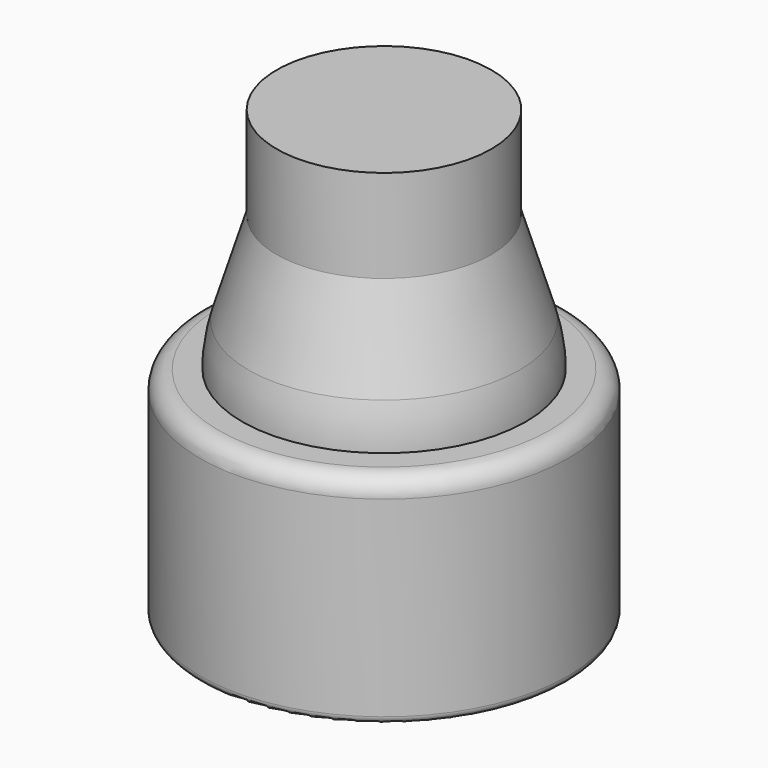
from build123d import *

# Parameters (mm, degrees)
F2_R     = 2.9977857905
F3_DEPTH = 5.85
F4_R     = 2.8
F5_DEPTH = 1
F5_TAPER = 70


# Not quite as in the source:
# - an extrude ends at something that could not be found from the text; its depth is read off the source's solid


with BuildPart() as f1:
    # F0 (on Front) → F1 (revolve)
    with BuildSketch(Plane.XZ):
        with BuildLine():
            Line((4.45, 5.85), (2.8, 5.85))
            Line((2.8, 5.85), (2.8, 3.65))
            Line((2.8, 3.65), (0.5, 2.3220943809))
            Line((0.5, 2.3220943809), (0, 2.3220943809))
            Line((0, 2.3220943809), (0, 0))
            Line((0, 0), (4.75, 0))
            ThreePointArc((4.75, 0), (4.8914213562, 0.0585786438), (4.95, 0.2))
            Line((4.95, 0.2), (4.95, 5.35))
            ThreePointArc((4.95, 5.35), (4.8035533906, 5.7035533906), (4.45, 5.85))
        make_face()
    revolve(axis=Axis((0, 0, 1.1610471904), (0, 0, -1)))

    # F2 (on face) → F3 (join, through all)
    with BuildSketch(Plane.XY.offset(5.85)):
        Circle(F2_R)
        with BuildLine():
            ThreePointArc((-0.5409184627, 2.3849386653), (0, 2.8), (0.5409184627, 2.3849386653))
            Line((0.5409184627, 2.3849386653), (0.5522855855, 2.3425159855))
            ThreePointArc((0.5522855855, 2.3425159855), (1.0088928953, 1.747453754), (1.7525355595, 1.6495513399))
            Line((1.7525355595, 1.6495513399), (1.7949582392, 1.6609184627))
            ThreePointArc((1.7949582392, 1.6609184627), (2.4248711306, 1.4), (2.3358767019, 0.7240202025))
            Line((2.3358767019, 0.7240202025), (2.304821145, 0.6929646456))
            ThreePointArc((2.304821145, 0.6929646456), (2.0177857905, 0), (2.304821145, -0.6929646456))
            Line((2.304821145, -0.6929646456), (2.3358767019, -0.7240202025))
            ThreePointArc((2.3358767019, -0.7240202025), (2.4248711306, -1.4), (1.7949582392, -1.6609184627))
            Line((1.7949582392, -1.6609184627), (1.7525355595, -1.6495513399))
            ThreePointArc((1.7525355595, -1.6495513399), (1.0088928953, -1.747453754), (0.5522855855, -2.3425159855))
            Line((0.5522855855, -2.3425159855), (0.5409184627, -2.3849386653))
            ThreePointArc((0.5409184627, -2.3849386653), (0, -2.8), (-0.5409184627, -2.3849386653))
            Line((-0.5409184627, -2.3849386653), (-0.5522855855, -2.3425159855))
            ThreePointArc((-0.5522855855, -2.3425159855), (-1.0088928953, -1.747453754), (-1.7525355595, -1.6495513399))
            Line((-1.7525355595, -1.6495513399), (-1.7949582392, -1.6609184627))
            ThreePointArc((-1.7949582392, -1.6609184627), (-2.4248711306, -1.4), (-2.3358767019, -0.7240202025))
            Line((-2.3358767019, -0.7240202025), (-2.304821145, -0.6929646456))
            ThreePointArc((-2.304821145, -0.6929646456), (-2.0177857905, 0), (-2.304821145, 0.6929646456))
            Line((-2.304821145, 0.6929646456), (-2.3358767019, 0.7240202025))
            ThreePointArc((-2.3358767019, 0.7240202025), (-2.4248711306, 1.4), (-1.7949582392, 1.6609184627))
            Line((-1.7949582392, 1.6609184627), (-1.7525355595, 1.6495513399))
            ThreePointArc((-1.7525355595, 1.6495513399), (-1.0088928953, 1.747453754), (-0.5522855855, 2.3425159855))
            Line((-0.5522855855, 2.3425159855), (-0.5409184627, 2.3849386653))
        make_face(mode=Mode.SUBTRACT)
    extrude(amount=-F3_DEPTH)

    # F4 (on face) → F5 (cut)
    with BuildSketch(Plane.XY.offset(5.85)):
        Circle(F4_R)
    extrude(amount=-F5_DEPTH, taper=F5_TAPER, mode=Mode.SUBTRACT)


with BuildPart() as f7:
    # F6 (on Front) → F7 (revolve)
    with BuildSketch(Plane.XZ):
        with BuildLine():
            Line((2.885, 12), (0, 12))
            Line((0, 12), (0, 0))
            Line((0, 0), (2.575, 0))
            Line((2.575, 0), (3.7168908213, 4.9460725434))
            ThreePointArc((3.7168908213, 4.9460725434), (3.8169738702, 5.9854747476), (3.644629586, 7.0153635796))
            Line((3.644629586, 7.0153635796), (2.885, 9.5))
            Line((2.885, 9.5), (2.885, 12))
        make_face()
    revolve(axis=Axis((0, 0, 6), (0, 0, -1)))


with BuildPart() as f9:
    # F8 (on Front) → F9 (revolve)
    with BuildSketch(Plane.XZ):
        with BuildLine():
            Line((0, 5.4649787367), (0, 0))
            Line((0, 0), (4.2405382264, 0))
            ThreePointArc((4.2405382264, 0), (4.4451377344, 0.0805938895), (4.5398074415, 0.2790730579))
            Line((4.5398074415, 0.2790730579), (4.8180895357, 4.2586924134))
            ThreePointArc((4.8180895357, 4.2586924134), (4.8318050114, 4.781163267), (4.8, 5.3028454963))
            ThreePointArc((4.8, 5.3028454963), (4.6437723065, 5.6163433494), (4.3201751845, 5.7504063897))
            Line((4.3201751845, 5.7504063897), (2.9, 5.8))
            Line((2.9, 5.8), (1, 5.4649787367))
            Line((1, 5.4649787367), (0, 5.4649787367))
        make_face()
    revolve(axis=Axis((0, 0, 2.7324893683), (0, 0, 1)))


solid = Compound([f1.part, f7.part, f9.part])
